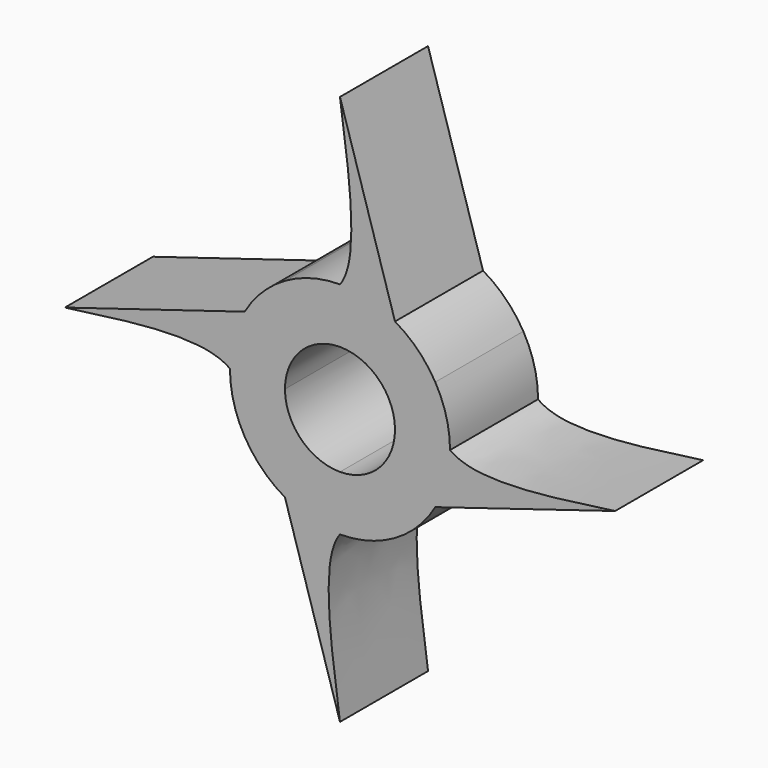
from build123d import *

# Parameters (mm, degrees)
F1_DEPTH = 10


# Not quite as in the source:
# - a feature names something its author has since deleted; it is built from what else it names


with BuildPart() as f1:
    # F0 (on Front) → F1 (new body)
    with BuildSketch(Plane.XZ):
        with BuildLine():
            add(Edge.make_bspline(
                [(10, 0), (8.6317372981, 1.0499048978), (8.645995668, 3.0249524489), (8.6602540378, 5)],
                knots=[0.6299429387, 0.6299429387, 0.6299429387, 0.6299429387, 1, 1, 1, 1], degree=3))
            ThreePointArc((10, 0), (9.6592582629, 2.588190451), (8.6602540378, 5))
        make_face()
        with BuildLine():
            add(Edge.make_bspline(
                [(25, 0), (18.6645871914, -0.8936191818), (12.3291743827, -1.7872383636), (10, 0)],
                knots=[0, 0, 0, 0, 0.6299429387, 0.6299429387, 0.6299429387, 0.6299429387], degree=3))
            ThreePointArc((10, 0), (9.6592582629, -2.588190451), (8.6602540378, -5))
            Line((8.6602540378, -5), (25, 0))
        make_face()
        with BuildLine():
            ThreePointArc((8.6602540378, -5), (9.6592582629, -2.588190451), (10, 0))
            Line((10, 0), (5, 0))
            Line((5, 0), (5, -4.9574967987))
            Line((5, -4.9574967987), (5, -5))
            Line((5, -5), (8.6602540378, -5))
        make_face()
        with BuildLine():
            Line((5, 0), (10, 0))
            add(Edge.make_bspline(
                [(10, 0), (8.6317372981, 1.0499048978), (8.645995668, 3.0249524489), (8.6602540378, 5)],
                knots=[0.6299429387, 0.6299429387, 0.6299429387, 0.6299429387, 1, 1, 1, 1], degree=3))
            Line((8.6602540378, 5), (5, 5))
            Line((5, 5), (5, 0))
        make_face()
        with BuildLine():
            Line((5, 5), (8.6602540378, 5))
            ThreePointArc((8.6602540378, 5), (7.0710678119, 7.0710678119), (5, 8.6602540378))
            Line((5, 8.6602540378), (5, 5))
        make_face()
        with BuildLine():
            ThreePointArc((5, -8.6602540378), (7.0710678119, -7.0710678119), (8.6602540378, -5))
            Line((8.6602540378, -5), (5, -5))
            Line((5, -5), (5, -8.6602540378))
        make_face()
        with BuildLine():
            ThreePointArc((0, 5), (3.5355339059, 3.5355339059), (5, 0))
            Line((5, 0), (5, 5))
            Line((5, 5), (4.9574967987, 5))
            Line((4.9574967987, 5), (0, 5))
        make_face()
        with BuildLine():
            Line((5, -4.9574967987), (5, 0))
            ThreePointArc((5, 0), (3.5355339059, -3.5355339059), (0, -5))
            Line((0, -5), (4.9574967987, -5))
            Line((4.9574967987, -5), (5, -5))
            Line((5, -5), (5, -4.9574967987))
        make_face()
        with BuildLine():
            Line((5, 5), (5, 8.6602540378))
            ThreePointArc((5, 8.6602540378), (2.588190451, 9.6592582629), (0, 10))
            Line((0, 10), (0, 5))
            Line((0, 5), (4.9574967987, 5))
            Line((4.9574967987, 5), (5, 5))
        make_face()
        with BuildLine():
            ThreePointArc((0, 10), (2.588190451, 9.6592582629), (5, 8.6602540378))
            Line((5, 8.6602540378), (0, 25))
            add(Edge.make_bspline(
                [(0, 25), (0.8936191818, 18.6645871914), (1.7872383636, 12.3291743827), (0, 10)],
                knots=[0, 0, 0, 0, 0.6299429387, 0.6299429387, 0.6299429387, 0.6299429387], degree=3))
        make_face()
        with BuildLine():
            add(Edge.make_bspline(
                [(0, -10), (1.0499048978, -8.6317372981), (3.0249524489, -8.645995668), (5, -8.6602540378)],
                knots=[0.6299429387, 0.6299429387, 0.6299429387, 0.6299429387, 1, 1, 1, 1], degree=3))
            Line((5, -8.6602540378), (5, -5))
            Line((5, -5), (4.9574967987, -5))
            Line((4.9574967987, -5), (0, -5))
            Line((0, -5), (0, -10))
        make_face()
        with BuildLine():
            ThreePointArc((0, -10), (2.588190451, -9.6592582629), (5, -8.6602540378))
            add(Edge.make_bspline(
                [(0, -10), (1.0499048978, -8.6317372981), (3.0249524489, -8.645995668), (5, -8.6602540378)],
                knots=[0.6299429387, 0.6299429387, 0.6299429387, 0.6299429387, 1, 1, 1, 1], degree=3))
        make_face()
        with BuildLine():
            Line((-5, 5), (0, 5))
            Line((0, 5), (0, 10))
            add(Edge.make_bspline(
                [(0, 10), (-1.0499048978, 8.6317372981), (-3.0249524489, 8.645995668), (-5, 8.6602540378)],
                knots=[0.6299429387, 0.6299429387, 0.6299429387, 0.6299429387, 1, 1, 1, 1], degree=3))
            Line((-5, 8.6602540378), (-5, 5))
        make_face()
        with BuildLine():
            ThreePointArc((-5, 0), (-3.5355339059, 3.5355339059), (0, 5))
            Line((0, 5), (-5, 5))
            Line((-5, 5), (-5, 0))
        make_face()
        with BuildLine():
            Line((0, -10), (0, -5))
            Line((0, -5), (-5, -5))
            Line((-5, -5), (-5, -8.6602540378))
            ThreePointArc((-5, -8.6602540378), (-2.588190451, -9.6592582629), (0, -10))
        make_face()
        with BuildLine():
            Line((-5, -5), (0, -5))
            ThreePointArc((0, -5), (-3.5355339059, -3.5355339059), (-5, 0))
            Line((-5, 0), (-5, -4.9574967987))
            Line((-5, -4.9574967987), (-5, -5))
        make_face()
        with BuildLine():
            add(Edge.make_bspline(
                [(0, 10), (-1.0499048978, 8.6317372981), (-3.0249524489, 8.645995668), (-5, 8.6602540378)],
                knots=[0.6299429387, 0.6299429387, 0.6299429387, 0.6299429387, 1, 1, 1, 1], degree=3))
            ThreePointArc((0, 10), (-2.588190451, 9.6592582629), (-5, 8.6602540378))
        make_face()
        with BuildLine():
            add(Edge.make_bspline(
                [(0, -25), (-0.8936191818, -18.6645871914), (-1.7872383636, -12.3291743827), (0, -10)],
                knots=[0, 0, 0, 0, 0.6299429387, 0.6299429387, 0.6299429387, 0.6299429387], degree=3))
            ThreePointArc((0, -10), (-2.588190451, -9.6592582629), (-5, -8.6602540378))
            Line((-5, -8.6602540378), (0, -25))
        make_face()
        with BuildLine():
            Line((-5, -4.9574967987), (-5, 0))
            Line((-5, 0), (-10, 0))
            add(Edge.make_bspline(
                [(-10, 0), (-8.6317383367, -1.0514075248), (-8.6459961873, -3.0257037624), (-8.6602540378, -5)],
                knots=[0.6299429387, 0.6299429387, 0.6299429387, 0.6299429387, 1, 1, 1, 1], degree=3))
            Line((-8.6602540378, -5), (-5, -5))
            Line((-5, -5), (-5, -4.9574967987))
        make_face()
        with BuildLine():
            Line((-10, 0), (-5, 0))
            Line((-5, 0), (-5, 5))
            Line((-5, 5), (-8.6602540378, 5))
            ThreePointArc((-8.6602540378, 5), (-9.6592582629, 2.588190451), (-10, 0))
        make_face()
        with BuildLine():
            Line((-8.6602540378, 5), (-5, 5))
            Line((-5, 5), (-5, 8.6602540378))
            ThreePointArc((-5, 8.6602540378), (-7.0710678119, 7.0710678119), (-8.6602540378, 5))
        make_face()
        with BuildLine():
            Line((-5, -8.6602540378), (-5, -5))
            Line((-5, -5), (-8.6602540378, -5))
            ThreePointArc((-8.6602540378, -5), (-7.0710678119, -7.0710678119), (-5, -8.6602540378))
        make_face()
        with BuildLine():
            add(Edge.make_bspline(
                [(-24.9999856665, 0.0207365385), (-18.6645791406, 0.9052664015), (-12.3291726147, 1.7897962644), (-10, 0)],
                knots=[0, 0, 0, 0, 0.6299429387, 0.6299429387, 0.6299429387, 0.6299429387], degree=3))
            ThreePointArc((-10, 0), (-9.6592582629, 2.588190451), (-8.6602540378, 5))
            Line((-8.6602540378, 5), (-24.9999856665, 0.0207365385))
        make_face()
        with BuildLine():
            add(Edge.make_bspline(
                [(-10, 0), (-8.6317383367, -1.0514075248), (-8.6459961873, -3.0257037624), (-8.6602540378, -5)],
                knots=[0.6299429387, 0.6299429387, 0.6299429387, 0.6299429387, 1, 1, 1, 1], degree=3))
            ThreePointArc((-10, 0), (-9.6592582629, -2.588190451), (-8.6602540378, -5))
        make_face()
    extrude(amount=F1_DEPTH)


solid = f1.part
